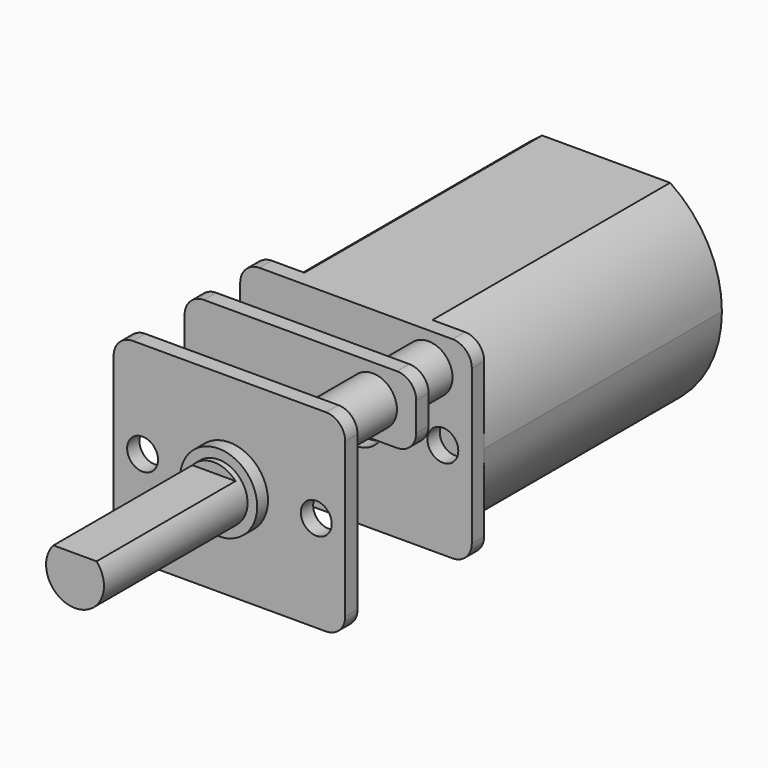
from build123d import *

# Parameters (mm, degrees)
F1_DEPTH      = 15.4
F3_DEPTH      = 0.8
F4_DEPTH      = 1.8
F5_R          = 0.8
F5_R_2        = 1.5
F6_DEPTH      = 9
F7_W          = 3.8
F7_H          = 10
F7_W_2        = 2.8
F8_DEPTH      = 25
F8_DEPTH_BACK = 25
F10_DEPTH     = 1
F12_R         = 1.25
F13_DEPTH     = 7.4
F15_R         = 2
F16_DEPTH     = 0.7
F17_DEPTH     = 1
F18_DEPTH     = 10


with BuildPart() as f1:
    # F0 (on Front) → F1 (new body)
    with BuildSketch(Plane.XZ):
        with BuildLine():
            ThreePointArc((3.3166247904, -5), (5.2867640737, -2.8372743309), (6, 0))
            ThreePointArc((6, 0), (5.2867640737, 2.8372743309), (3.3166247904, 5))
            Line((3.3166247904, 5), (-3.3166247904, 5))
            ThreePointArc((-3.3166247904, 5), (-5.2867640737, 2.8372743309), (-6, 0))
            ThreePointArc((-6, 0), (-5.2867640737, -2.8372743309), (-3.3166247904, -5))
            Line((-3.3166247904, -5), (3.3166247904, -5))
        make_face()
    extrude(amount=F1_DEPTH)

    # F2 (on Front) → F3 (join)
    with BuildSketch(Plane.XZ):
        with BuildLine():
            Line((2.5, 0), (-2.5, 0))
            ThreePointArc((-2.5, 0), (0, -2.5), (2.5, 0))
        make_face()
        with BuildLine():
            ThreePointArc((2.5, 0), (0, 2.5), (-2.5, 0))
            Line((-2.5, 0), (2.5, 0))
        make_face()
    extrude(amount=-F3_DEPTH)

    # F2 (on Front) → F4 (join)
    with BuildSketch(Plane.XZ):
        Polygon((3, 1), (3, 0), (3, -1), (3.2, -1), (3.2, 1), align=None)
        Polygon((-3, 1), (-3.2, 1), (-3.2, -1), (-3, -1), (-3, 0), align=None)
    extrude(amount=-F4_DEPTH)

    # F5 (on face) → F6 (join)
    with BuildSketch(Plane.XZ.offset(15.4)):
        with BuildLine():
            Line((5, 5), (-5, 5))
            ThreePointArc((-5, 5), (-5.7071067812, 4.7071067812), (-6, 4))
            Line((-6, 4), (-6, -4))
            ThreePointArc((-6, -4), (-5.7071067812, -4.7071067812), (-5, -5))
            Line((-5, -5), (5, -5))
            ThreePointArc((5, -5), (5.7071067812, -4.7071067812), (6, -4))
            Line((6, -4), (6, 4))
            ThreePointArc((6, 4), (5.7071067812, 4.7071067812), (5, 5))
        make_face()
        with Locations((-4.5, 0)):
            Circle(F5_R, mode=Mode.SUBTRACT)
        Circle(F5_R_2, mode=Mode.SUBTRACT)
        with Locations((4.5, 0)):
            Circle(F5_R, mode=Mode.SUBTRACT)
    extrude(amount=F6_DEPTH)

    # F7 (on Right) → F8 (cut, two sides)
    with BuildSketch(Plane.YZ) as f8_sk:
        with Locations((-21.7, 0)):
            Rectangle(F7_W, F7_H)
        with Locations((-17.6, 0)):
            Rectangle(F7_W_2, F7_H)
    extrude(amount=-F8_DEPTH, mode=Mode.SUBTRACT)
    extrude(f8_sk.sketch, amount=F8_DEPTH_BACK, mode=Mode.SUBTRACT)

    # F9 (on face) → F10 (cut)
    with BuildSketch(Plane.XZ.offset(19.8)):
        with BuildLine():
            Line((5, 1.5), (0, 1.5))
            ThreePointArc((0, 1.5), (-1.0606601718, 1.0606601718), (-1.5, 0))
            Line((-1.5, 0), (-1.5, -4))
            ThreePointArc((-1.5, -4), (-1.7928932188, -4.7071067812), (-2.5, -5))
            Line((-2.5, -5), (-2.5, -6))
            Line((-2.5, -6), (-1.5, -6))
            Line((-1.5, -6), (7, -6))
            Line((7, -6), (7, 2.5))
            Line((7, 2.5), (6, 2.5))
            ThreePointArc((6, 2.5), (5.7071067812, 1.7928932188), (5, 1.5))
        make_face()
    extrude(amount=-F10_DEPTH, mode=Mode.SUBTRACT)

    # F12 (on offset) → F13 (join)
    with BuildSketch(Plane.XZ.offset(16.2)):
        with Locations((-3.75, -3.25)):
            Circle(F12_R)
        with Locations((3.75, 3.25)):
            Circle(F12_R)
    extrude(amount=F13_DEPTH)

    # F15 (on offset) → F16 (join)
    with BuildSketch(Plane.XZ.offset(24.4)):
        Circle(F15_R)
        with BuildLine():
            ThreePointArc((1.1180339887, 1), (1.4012585384, 0.5352331347), (1.5, 0))
            ThreePointArc((1.5, 0), (-0.5352331347, -1.4012585384), (-1.1180339887, 1))
            ThreePointArc((-1.1180339887, 1), (0, 1.5), (1.1180339887, 1))
        make_face(mode=Mode.SUBTRACT)
    extrude(amount=F16_DEPTH)

    # F15 (on offset) → F17 (join)
    with BuildSketch(Plane.XZ.offset(24.4)):
        with BuildLine():
            Line((-1.1180339887, 1), (1.1180339887, 1))
            ThreePointArc((1.1180339887, 1), (0, 1.5), (-1.1180339887, 1))
        make_face()
        with BuildLine():
            ThreePointArc((-1.1180339887, 1), (-0.5352331347, -1.4012585384), (1.5, 0))
            ThreePointArc((1.5, 0), (1.4012585384, 0.5352331347), (1.1180339887, 1))
            Line((1.1180339887, 1), (-1.1180339887, 1))
        make_face()
    extrude(amount=F17_DEPTH)

    # F15 (on offset) → F18 (join)
    with BuildSketch(Plane.XZ.offset(24.4)):
        with BuildLine():
            ThreePointArc((-1.1180339887, 1), (-0.5352331347, -1.4012585384), (1.5, 0))
            ThreePointArc((1.5, 0), (1.4012585384, 0.5352331347), (1.1180339887, 1))
            Line((1.1180339887, 1), (-1.1180339887, 1))
        make_face()
    extrude(amount=F18_DEPTH)


solid = f1.part
